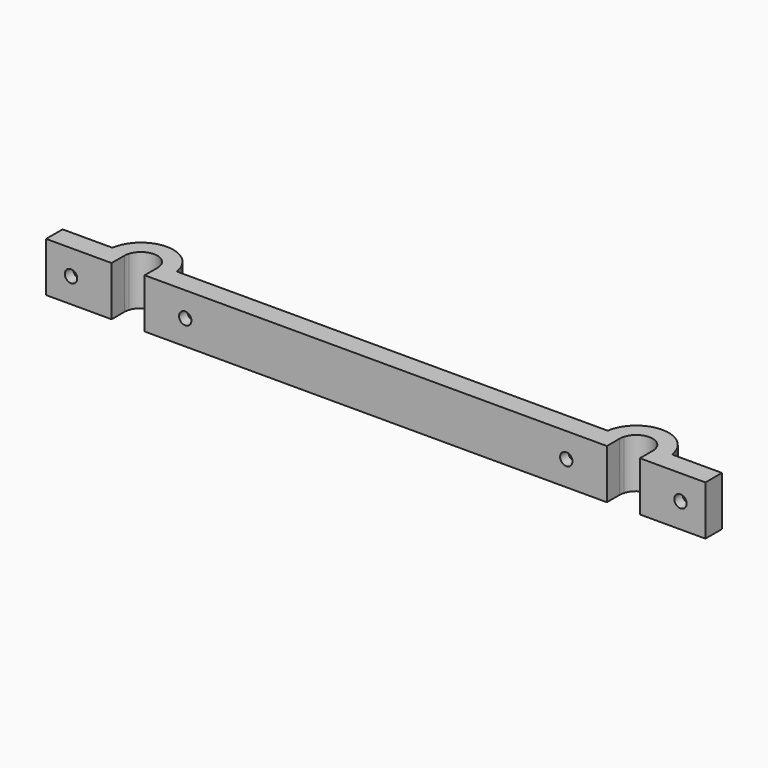
from build123d import *

# Parameters (mm, degrees)
F0_W     = 3.875
F0_H     = 3.875
F1_DEPTH = 12
F3_DEPTH = 2.5
F4_R     = 1.5
F5_DEPTH = 5.001


# Not quite as in the source:
# - a pattern or mirror of a feature is missing from the dataset's text; its kind, count and spacing are read off the source's solid
# - a feature names something its author has since deleted; it is built from what else it names


with BuildPart() as f1:
    # F0 (on Top) → F1 (new body)
    with BuildSketch(Plane.XY):
        with BuildLine():
            Line((-67.7942286341, 5), (-79.875, 5))
            Line((-79.875, 5), (-79.875, 0))
            Line((-79.875, 0), (-67.875, 0))
            Line((-67.875, 0), (-67.875, 3.875))
            ThreePointArc((-67.875, 3.875), (-67.854781203, 4.4389479173), (-67.7942286341, 5))
        make_face()
        with BuildLine():
            ThreePointArc((-52.2057713659, 5), (-60, 11.75), (-67.7942286341, 5))
            Line((-67.7942286341, 5), (-63.8385381332, 5))
            ThreePointArc((-63.8385381332, 5), (-60, 7.875), (-56.1614618668, 5))
            Line((-56.1614618668, 5), (-52.2057713659, 5))
        make_face()
        with BuildLine():
            Line((-63.8385381332, 5), (-67.7942286341, 5))
            ThreePointArc((-67.7942286341, 5), (-67.854781203, 4.4389479173), (-67.875, 3.875))
            Line((-67.875, 3.875), (-64, 3.875))
            ThreePointArc((-64, 3.875), (-63.9594287803, 4.4432637888), (-63.8385381332, 5))
        make_face()
        with BuildLine():
            ThreePointArc((-52.125, 3.875), (-52.145218797, 4.4389479173), (-52.2057713659, 5))
            Line((-52.2057713659, 5), (-56.1614618668, 5))
            ThreePointArc((-56.1614618668, 5), (-56.0405712197, 4.4432637888), (-56, 3.875))
            Line((-56, 3.875), (-52.125, 3.875))
        make_face()
        with BuildLine():
            Line((52.2057713659, 5), (-52.2057713659, 5))
            ThreePointArc((-52.2057713659, 5), (-52.145218797, 4.4389479173), (-52.125, 3.875))
            Line((-52.125, 3.875), (-52.125, 0))
            Line((-52.125, 0), (52.125, 0))
            Line((52.125, 0), (52.125, 3.875))
            ThreePointArc((52.125, 3.875), (52.145218797, 4.4389479173), (52.2057713659, 5))
        make_face()
        with Locations((-65.9375, 1.9375)):
            Rectangle(F0_W, F0_H)
        with BuildLine():
            ThreePointArc((67.7942286341, 5), (60, 11.75), (52.2057713659, 5))
            Line((52.2057713659, 5), (56.1614618668, 5))
            ThreePointArc((56.1614618668, 5), (60, 7.875), (63.8385381332, 5))
            Line((63.8385381332, 5), (67.7942286341, 5))
        make_face()
        with BuildLine():
            Line((56.1614618668, 5), (52.2057713659, 5))
            ThreePointArc((52.2057713659, 5), (52.145218797, 4.4389479173), (52.125, 3.875))
            Line((52.125, 3.875), (56, 3.875))
            ThreePointArc((56, 3.875), (56.0405712197, 4.4432637888), (56.1614618668, 5))
        make_face()
        with Locations((-54.0625, 1.9375)):
            Rectangle(F0_W, F0_H)
        with BuildLine():
            ThreePointArc((67.875, 3.875), (67.854781203, 4.4389479173), (67.7942286341, 5))
            Line((67.7942286341, 5), (63.8385381332, 5))
            ThreePointArc((63.8385381332, 5), (63.9594287803, 4.4432637888), (64, 3.875))
            Line((64, 3.875), (67.875, 3.875))
        make_face()
        with BuildLine():
            Line((79.875, 5), (67.7942286341, 5))
            ThreePointArc((67.7942286341, 5), (67.854781203, 4.4389479173), (67.875, 3.875))
            Line((67.875, 3.875), (67.875, 0))
            Line((67.875, 0), (79.875, 0))
            Line((79.875, 0), (79.875, 5))
        make_face()
        with Locations((54.0625, 1.9375)):
            Rectangle(F0_W, F0_H)
        with Locations((65.9375, 1.9375)):
            Rectangle(F0_W, F0_H)
    extrude(amount=F1_DEPTH)

    # F2 (on face) → F3 (cut)
    with BuildSketch(Plane(origin=(0, 5, 0), x_dir=(-1, 0, 0), z_dir=(0, 1, 0))):
        Polygon((44.2745635514, 2.725), (48.0562078146, 2.725), (49.9470299462, 6), (48.0562078146, 9.275), (44.2745635514, 9.275), (42.3837414198, 6), align=None)
        Polygon((71.9437921854, 2.725), (75.7254364486, 2.725), (77.6162585802, 6), (75.7254364486, 9.275), (71.9437921854, 9.275), (70.0529700538, 6), align=None)
    f3 = extrude(amount=-F3_DEPTH, mode=Mode.SUBTRACT)

    # F3_copies: F3 across plane
    add(f3.mirror(Plane(origin=(0, 0, 0), x_dir=(0, 0, 1), z_dir=(1, 0, 0))), mode=Mode.SUBTRACT)

    # F4 (on face) → F5 (cut, through all)
    with BuildSketch(Plane(origin=(0, 5, 0), x_dir=(-1, 0, 0), z_dir=(0, 1, 0))):
        with Locations((46.165385683, 6)):
            Circle(F4_R)
        with Locations((73.834614317, 6)):
            Circle(F4_R)
    f5 = extrude(amount=-F5_DEPTH, mode=Mode.SUBTRACT)

    # F5_copies: F5 across plane
    add(f5.mirror(Plane(origin=(0, 0, 0), x_dir=(0, 0, 1), z_dir=(1, 0, 0))), mode=Mode.SUBTRACT)


solid = f1.part
